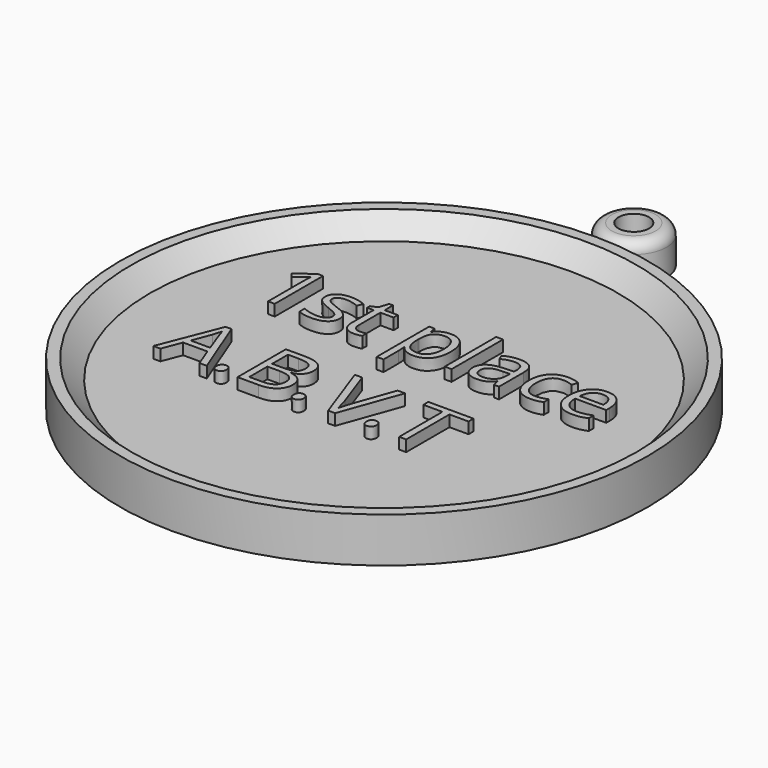
from build123d import *

# Parameters (mm, degrees)
F0_R         = 44.7882725857
F0_R_2       = 37.8315879498
F1_DEPTH     = 7.62
F0_R_3       = 5.569727431
F0_R_4       = 2.5947856339
F2_DEPTH     = 6.35
F3_R         = 1.8396307345
F0_W         = 1.1629488242
F0_H         = 10.8967632599
F4_DEPTH     = 4.445
F0_TEXT_SIZE = 14.3407947487
F5_DEPTH     = 6.35


# Not quite as in the source:
# - a fillet or chamfer that OpenCascade refuses, or shapes differently, is made with other operations: its cross-section is extruded or revolved along the edge and cut away or added
# - Text() gives the source's letters only with a copy of the font that has no kerning and outlines rounded to 1/6400 em; it was checked with that copy


with BuildPart() as f1:
    # F0 (on Top) → F1 (new body)
    with BuildSketch(Plane.XY):
        with Locations((-31.6393449903, -5.1120719872)):
            Circle(F0_R)
        with Locations((-31.6393449903, -5.1120719872)):
            Circle(F0_R_2, mode=Mode.SUBTRACT)
    extrude(amount=F1_DEPTH)

    # F0 (on Top) → F4 (join)
    with BuildSketch(Plane.XY):
        with Locations((-31.6393449903, -5.1120719872)):
            Circle(F0_R_2)
        Polygon((-50.1972631189, -19.5034808583), (-51.4296751676, -19.5034808583), (-52.7046614508, -16.2476723005), (-56.8074731984, -16.2476723005), (-58.0667742373, -19.5034808583), (-59.2722972958, -19.5034808583), (-55.2255042777, -9.2229236228), (-54.2238893945, -9.2229236228), align=None, mode=Mode.SUBTRACT)
        with BuildLine():
            add(Edge.make_bspline(
                [(-48.8987489694, -19.4866752394), (-49.1329072587, -19.2659614452), (-49.1329072587, -18.7617928799)],
                knots=[0, 0, 0, 1, 1, 1], degree=2))
            add(Edge.make_bspline(
                [(-49.1329072587, -18.7617928799), (-49.1329072587, -18.2912355522), (-48.918915712, -18.0503550154)],
                knots=[0, 0, 0, 1, 1, 1], degree=2))
            add(Edge.make_bspline(
                [(-48.918915712, -18.0503550154), (-48.7049241654, -17.8094744786), (-48.3060708114, -17.8094744786)],
                knots=[0, 0, 0, 1, 1, 1], degree=2))
            add(Edge.make_bspline(
                [(-48.3060708114, -17.8094744786), (-47.9004952099, -17.8094744786), (-47.6730591682, -18.0503550154)],
                knots=[0, 0, 0, 1, 1, 1], degree=2))
            add(Edge.make_bspline(
                [(-47.6730591682, -18.0503550154), (-47.4456231265, -18.2912355522), (-47.4456231265, -18.7617928799)],
                knots=[0, 0, 0, 1, 1, 1], degree=2))
            add(Edge.make_bspline(
                [(-47.4456231265, -18.7617928799), (-47.4456231265, -19.2166649633), (-47.676420292, -19.4620269985)],
                knots=[0, 0, 0, 1, 1, 1], degree=2))
            add(Edge.make_bspline(
                [(-47.676420292, -19.4620269985), (-47.9072174575, -19.7073890336), (-48.3060708114, -19.7073890336)],
                knots=[0, 0, 0, 1, 1, 1], degree=2))
            add(Edge.make_bspline(
                [(-48.3060708114, -19.7073890336), (-48.6645906801, -19.7073890336), (-48.8987489694, -19.4866752394)],
                knots=[0, 0, 0, 1, 1, 1], degree=2))
        make_face(mode=Mode.SUBTRACT)
        with BuildLine():
            add(Edge.make_bspline(
                [(-35.7903662694, -19.4866752394), (-36.0245245586, -19.2659614452), (-36.0245245586, -18.7617928799)],
                knots=[0, 0, 0, 1, 1, 1], degree=2))
            add(Edge.make_bspline(
                [(-36.0245245586, -18.7617928799), (-36.0245245586, -18.2912355522), (-35.810533012, -18.0503550154)],
                knots=[0, 0, 0, 1, 1, 1], degree=2))
            add(Edge.make_bspline(
                [(-35.810533012, -18.0503550154), (-35.5965414654, -17.8094744786), (-35.1976881114, -17.8094744786)],
                knots=[0, 0, 0, 1, 1, 1], degree=2))
            add(Edge.make_bspline(
                [(-35.1976881114, -17.8094744786), (-34.7921125099, -17.8094744786), (-34.5646764682, -18.0503550154)],
                knots=[0, 0, 0, 1, 1, 1], degree=2))
            add(Edge.make_bspline(
                [(-34.5646764682, -18.0503550154), (-34.3372404265, -18.2912355522), (-34.3372404265, -18.7617928799)],
                knots=[0, 0, 0, 1, 1, 1], degree=2))
            add(Edge.make_bspline(
                [(-34.3372404265, -18.7617928799), (-34.3372404265, -19.2166649633), (-34.568037592, -19.4620269985)],
                knots=[0, 0, 0, 1, 1, 1], degree=2))
            add(Edge.make_bspline(
                [(-34.568037592, -19.4620269985), (-34.7988347575, -19.7073890336), (-35.1976881114, -19.7073890336)],
                knots=[0, 0, 0, 1, 1, 1], degree=2))
            add(Edge.make_bspline(
                [(-35.1976881114, -19.7073890336), (-35.5562079801, -19.7073890336), (-35.7903662694, -19.4866752394)],
                knots=[0, 0, 0, 1, 1, 1], degree=2))
        make_face(mode=Mode.SUBTRACT)
        with BuildLine():
            Line((-44.9740767815, -19.5034808583), (-44.9740767815, -9.2654978572))
            Line((-44.9740767815, -9.2654978572), (-42.0812695908, -9.2654978572))
            add(Edge.make_bspline(
                [(-42.0812695908, -9.2654978572), (-40.0444285866, -9.2654978572), (-39.1335640452, -9.874981634)],
                knots=[0, 0, 0, 1, 1, 1], degree=2))
            add(Edge.make_bspline(
                [(-39.1335640452, -9.874981634), (-38.2226995037, -10.4844654108), (-38.2226995037, -11.7997851792)],
                knots=[0, 0, 0, 1, 1, 1], degree=2))
            add(Edge.make_bspline(
                [(-38.2226995037, -11.7997851792), (-38.2226995037, -12.7117700952), (-38.7302291929, -13.3033278786)],
                knots=[0, 0, 0, 1, 1, 1], degree=2))
            add(Edge.make_bspline(
                [(-38.7302291929, -13.3033278786), (-39.237758882, -13.894885662), (-40.2124847751, -14.069664098)],
                knots=[0, 0, 0, 1, 1, 1], degree=2))
            Line((-40.2124847751, -14.069664098), (-40.2124847751, -14.1391273226))
            add(Edge.make_bspline(
                [(-40.2124847751, -14.1391273226), (-37.8798648793, -14.5379806765), (-37.8798648793, -16.5905069249)],
                knots=[0, 0, 0, 1, 1, 1], degree=2))
            add(Edge.make_bspline(
                [(-37.8798648793, -16.5905069249), (-37.8798648793, -17.9618454228), (-38.8075350396, -18.7326631405)],
                knots=[0, 0, 0, 1, 1, 1], degree=2))
            add(Edge.make_bspline(
                [(-38.8075350396, -18.7326631405), (-39.7352051999, -19.5034808583), (-41.4023225894, -19.5034808583)],
                knots=[0, 0, 0, 1, 1, 1], degree=2))
            Line((-41.4023225894, -19.5034808583), (-44.9740767815, -19.5034808583))
        make_face(mode=Mode.SUBTRACT)
        with BuildLine():
            add(Edge.make_bspline(
                [(-23.439356792, -19.4866752394), (-23.6735150813, -19.2659614452), (-23.6735150813, -18.7617928799)],
                knots=[0, 0, 0, 1, 1, 1], degree=2))
            add(Edge.make_bspline(
                [(-23.6735150813, -18.7617928799), (-23.6735150813, -18.2912355522), (-23.4595235347, -18.0503550154)],
                knots=[0, 0, 0, 1, 1, 1], degree=2))
            add(Edge.make_bspline(
                [(-23.4595235347, -18.0503550154), (-23.245531988, -17.8094744786), (-22.8466786341, -17.8094744786)],
                knots=[0, 0, 0, 1, 1, 1], degree=2))
            add(Edge.make_bspline(
                [(-22.8466786341, -17.8094744786), (-22.4411030326, -17.8094744786), (-22.2136669909, -18.0503550154)],
                knots=[0, 0, 0, 1, 1, 1], degree=2))
            add(Edge.make_bspline(
                [(-22.2136669909, -18.0503550154), (-21.9862309491, -18.2912355522), (-21.9862309491, -18.7617928799)],
                knots=[0, 0, 0, 1, 1, 1], degree=2))
            add(Edge.make_bspline(
                [(-21.9862309491, -18.7617928799), (-21.9862309491, -19.2166649633), (-22.2170281146, -19.4620269985)],
                knots=[0, 0, 0, 1, 1, 1], degree=2))
            add(Edge.make_bspline(
                [(-22.2170281146, -19.4620269985), (-22.4478252801, -19.7073890336), (-22.8466786341, -19.7073890336)],
                knots=[0, 0, 0, 1, 1, 1], degree=2))
            add(Edge.make_bspline(
                [(-22.8466786341, -19.7073890336), (-23.2051985028, -19.7073890336), (-23.439356792, -19.4866752394)],
                knots=[0, 0, 0, 1, 1, 1], degree=2))
        make_face(mode=Mode.SUBTRACT)
        with BuildLine():
            Line((-28.3566808664, -15.8488189465), (-26.017338723, -9.2654978572))
            Line((-26.017338723, -9.2654978572), (-24.7378709416, -9.2654978572))
            Line((-24.7378709416, -9.2654978572), (-28.426144091, -19.5034808583))
            Line((-28.426144091, -19.5034808583), (-29.6025374102, -19.5034808583))
            Line((-29.6025374102, -19.5034808583), (-33.2728845662, -9.2654978572))
            Line((-33.2728845662, -9.2654978572), (-32.0113427782, -9.2654978572))
            Line((-32.0113427782, -9.2654978572), (-29.6585561397, -15.8891524318))
            add(Edge.make_bspline(
                [(-29.6585561397, -15.8891524318), (-29.2529805382, -17.0319345133), (-29.0154611252, -18.1097348686)],
                knots=[0, 0, 0, 1, 1, 1], degree=2))
            add(Edge.make_bspline(
                [(-29.0154611252, -18.1097348686), (-28.7622564679, -16.9759157838), (-28.3566808664, -15.8488189465)],
                knots=[0, 0, 0, 1, 1, 1], degree=2))
        make_face(mode=Mode.SUBTRACT)
        Polygon((-16.3641912578, -10.3231314699), (-16.3641912578, -19.5034808583), (-17.5540290721, -19.5034808583), (-17.5540290721, -10.3231314699), (-20.7963931348, -10.3231314699), (-20.7963931348, -9.2654978572), (-13.1218271951, -9.2654978572), (-13.1218271951, -10.3231314699), align=None, mode=Mode.SUBTRACT)
        with BuildLine():
            Line((-54.2664636289, 10.2379830011), (-54.2664636289, 0))
            Line((-54.2664636289, 0), (-55.4002827137, 0))
            Line((-55.4002827137, 0), (-55.4002827137, 7.2958793284))
            add(Edge.make_bspline(
                [(-55.4002827137, 7.2958793284), (-55.4002827137, 8.2078642445), (-55.3442639842, 9.0190154474)],
                knots=[0, 0, 0, 1, 1, 1], degree=2))
            add(Edge.make_bspline(
                [(-55.3442639842, 9.0190154474), (-55.4899126809, 8.8711260016), (-55.672533739, 8.7109124353)],
                knots=[0, 0, 0, 1, 1, 1], degree=2))
            add(Edge.make_bspline(
                [(-55.672533739, 8.7109124353), (-55.8551547971, 8.5506988689), (-57.3385307539, 7.3451758104)],
                knots=[0, 0, 0, 1, 1, 1], degree=2))
            Line((-57.3385307539, 7.3451758104), (-57.9547367783, 8.1428825183))
            Line((-57.9547367783, 8.1428825183), (-55.2456710203, 10.2379830011))
            Line((-55.2456710203, 10.2379830011), (-54.2664636289, 10.2379830011))
        make_face(mode=Mode.SUBTRACT)
        with BuildLine():
            add(Edge.make_bspline(
                [(-45.3706893863, 3.3611237692), (-44.8911690619, 2.8569552038), (-44.8911690619, 2.0928597336)],
                knots=[0, 0, 0, 1, 1, 1], degree=2))
            add(Edge.make_bspline(
                [(-44.8911690619, 2.0928597336), (-44.8911690619, 1.0217816258), (-45.6888757698, 0.4403072138)],
                knots=[0, 0, 0, 1, 1, 1], degree=2))
            add(Edge.make_bspline(
                [(-45.6888757698, 0.4403072138), (-46.4865824777, -0.1411671983), (-47.9296249493, -0.1411671983)],
                knots=[0, 0, 0, 1, 1, 1], degree=2))
            add(Edge.make_bspline(
                [(-47.9296249493, -0.1411671983), (-49.4555751405, -0.1411671983), (-50.3093005779, 0.3428346245)],
                knots=[0, 0, 0, 1, 1, 1], degree=2))
            Line((-50.3093005779, 0.3428346245), (-50.3093005779, 1.4206349798))
            add(Edge.make_bspline(
                [(-50.3093005779, 1.4206349798), (-49.7558355306, 1.1405413324), (-49.1228238873, 0.980327766)],
                knots=[0, 0, 0, 1, 1, 1], degree=2))
            add(Edge.make_bspline(
                [(-49.1228238873, 0.980327766), (-48.4898122441, 0.8201141997), (-47.9004952099, 0.8201141997)],
                knots=[0, 0, 0, 1, 1, 1], degree=2))
            add(Edge.make_bspline(
                [(-47.9004952099, 0.8201141997), (-46.9907510431, 0.8201141997), (-46.5011473473, 1.1102912184)],
                knots=[0, 0, 0, 1, 1, 1], degree=2))
            add(Edge.make_bspline(
                [(-46.5011473473, 1.1102912184), (-46.0115436516, 1.4004682372), (-46.0115436516, 1.9965075189)],
                knots=[0, 0, 0, 1, 1, 1], degree=2))
            add(Edge.make_bspline(
                [(-46.0115436516, 1.9965075189), (-46.0115436516, 2.4446573548), (-46.3991932597, 2.7628437383)],
                knots=[0, 0, 0, 1, 1, 1], degree=2))
            add(Edge.make_bspline(
                [(-46.3991932597, 2.7628437383), (-46.7868428677, 3.0810301218), (-47.9161804542, 3.5157354626)],
                knots=[0, 0, 0, 1, 1, 1], degree=2))
            add(Edge.make_bspline(
                [(-47.9161804542, 3.5157354626), (-48.987258562, 3.9145888166), (-49.4387695217, 4.2126084574)],
                knots=[0, 0, 0, 1, 1, 1], degree=2))
            add(Edge.make_bspline(
                [(-49.4387695217, 4.2126084574), (-49.8902804813, 4.5106280983), (-50.1109942755, 4.8881943351)],
                knots=[0, 0, 0, 1, 1, 1], degree=2))
            add(Edge.make_bspline(
                [(-50.1109942755, 4.8881943351), (-50.3317080697, 5.2657605718), (-50.3317080697, 5.7900958798)],
                knots=[0, 0, 0, 1, 1, 1], degree=2))
            add(Edge.make_bspline(
                [(-50.3317080697, 5.7900958798), (-50.3317080697, 6.728969786), (-49.5676125995, 7.272351462)],
                knots=[0, 0, 0, 1, 1, 1], degree=2))
            add(Edge.make_bspline(
                [(-49.5676125995, 7.272351462), (-48.8035171293, 7.8157331381), (-47.4747528658, 7.8157331381)],
                knots=[0, 0, 0, 1, 1, 1], degree=2))
            add(Edge.make_bspline(
                [(-47.4747528658, 7.8157331381), (-46.2356185696, 7.8157331381), (-45.0502622536, 7.3115645727)],
                knots=[0, 0, 0, 1, 1, 1], degree=2))
            Line((-45.0502622536, 7.3115645727), (-45.4648008518, 6.3659684189))
            add(Edge.make_bspline(
                [(-45.4648008518, 6.3659684189), (-46.6187866793, 6.841007245), (-47.5576605855, 6.841007245)],
                knots=[0, 0, 0, 1, 1, 1], degree=2))
            add(Edge.make_bspline(
                [(-47.5576605855, 6.841007245), (-48.3844970327, 6.841007245), (-48.8046375039, 6.5822007147)],
                knots=[0, 0, 0, 1, 1, 1], degree=2))
            add(Edge.make_bspline(
                [(-48.8046375039, 6.5822007147), (-49.224777975, 6.3233941845), (-49.224777975, 5.8685221011)],
                knots=[0, 0, 0, 1, 1, 1], degree=2))
            add(Edge.make_bspline(
                [(-49.224777975, 5.8685221011), (-49.224777975, 5.5592987143), (-49.0668051579, 5.3430664185)],
                knots=[0, 0, 0, 1, 1, 1], degree=2))
            add(Edge.make_bspline(
                [(-49.0668051579, 5.3430664185), (-48.9088323407, 5.1268341227), (-48.5592754687, 4.9307685695)],
                knots=[0, 0, 0, 1, 1, 1], degree=2))
            add(Edge.make_bspline(
                [(-48.5592754687, 4.9307685695), (-48.2097185967, 4.7347030163), (-47.214825961, 4.3627386525)],
                knots=[0, 0, 0, 1, 1, 1], degree=2))
            add(Edge.make_bspline(
                [(-47.214825961, 4.3627386525), (-45.8502097107, 3.8652923346), (-45.3706893863, 3.3611237692)],
                knots=[0, 0, 0, 1, 1, 1], degree=2))
        make_face(mode=Mode.SUBTRACT)
        with BuildLine():
            add(Edge.make_bspline(
                [(-41.4247300812, 1.1909581889), (-41.0953399518, 0.8201141997), (-40.5217081619, 0.8201141997)],
                knots=[0, 0, 0, 1, 1, 1], degree=2))
            add(Edge.make_bspline(
                [(-40.5217081619, 0.8201141997), (-40.2124847751, 0.8201141997), (-39.9256688801, 0.8649291833)],
                knots=[0, 0, 0, 1, 1, 1], degree=2))
            add(Edge.make_bspline(
                [(-39.9256688801, 0.8649291833), (-39.6388529852, 0.9097441669), (-39.4707967967, 0.9590406488)],
                knots=[0, 0, 0, 1, 1, 1], degree=2))
            Line((-39.4707967967, 0.9590406488), (-39.4707967967, 0.0694632246))
            add(Edge.make_bspline(
                [(-39.4707967967, 0.0694632246), (-39.6590197278, -0.0201667426), (-40.0265025932, -0.0806669705)],
                knots=[0, 0, 0, 1, 1, 1], degree=2))
            add(Edge.make_bspline(
                [(-40.0265025932, -0.0806669705), (-40.3939854586, -0.1411671983), (-40.6897643503, -0.1411671983)],
                knots=[0, 0, 0, 1, 1, 1], degree=2))
            add(Edge.make_bspline(
                [(-40.6897643503, -0.1411671983), (-42.9148282856, -0.1411671983), (-42.9148282856, 2.2048971926)],
                knots=[0, 0, 0, 1, 1, 1], degree=2))
            Line((-42.9148282856, 2.2048971926), (-42.9148282856, 6.7715440204))
            Line((-42.9148282856, 6.7715440204), (-44.0150361327, 6.7715440204))
            Line((-44.0150361327, 6.7715440204), (-44.0150361327, 7.3317313153))
            Line((-44.0150361327, 7.3317313153), (-42.9148282856, 7.8157331381))
            Line((-42.9148282856, 7.8157331381), (-42.4263449644, 9.4537207883))
            Line((-42.4263449644, 9.4537207883), (-41.7541202106, 9.4537207883))
            Line((-41.7541202106, 9.4537207883), (-41.7541202106, 7.6745659398))
            Line((-41.7541202106, 7.6745659398), (-39.5268155262, 7.6745659398))
            Line((-39.5268155262, 7.6745659398), (-39.5268155262, 6.7715440204))
            Line((-39.5268155262, 6.7715440204), (-41.7541202106, 6.7715440204))
            Line((-41.7541202106, 6.7715440204), (-41.7541202106, 2.2541936746))
            add(Edge.make_bspline(
                [(-41.7541202106, 2.2541936746), (-41.7541202106, 1.5618021781), (-41.4247300812, 1.1909581889)],
                knots=[0, 0, 0, 1, 1, 1], degree=2))
        make_face(mode=Mode.SUBTRACT)
        with BuildLine():
            add(Edge.make_bspline(
                [(-28.2973010132, 0.9063830431), (-29.1409430793, -0.1411671983), (-30.6400042803, -0.1411671983)],
                knots=[0, 0, 0, 1, 1, 1], degree=2))
            add(Edge.make_bspline(
                [(-30.6400042803, -0.1411671983), (-31.3906552555, -0.1411671983), (-32.0102224036, 0.1355653254)],
                knots=[0, 0, 0, 1, 1, 1], degree=2))
            add(Edge.make_bspline(
                [(-32.0102224036, 0.1355653254), (-32.6297895517, 0.412297849), (-33.0488096483, 0.9881703882)],
                knots=[0, 0, 0, 1, 1, 1], degree=2))
            Line((-33.0488096483, 0.9881703882), (-33.1339581171, 0.9881703882))
            add(Edge.make_bspline(
                [(-33.1339581171, 0.9881703882), (-33.0488096483, 0.3159456343), (-33.0488096483, -0.286815895)],
                knots=[0, 0, 0, 1, 1, 1], degree=2))
            Line((-33.0488096483, -0.286815895), (-33.0488096483, -3.4462722381))
            Line((-33.0488096483, -3.4462722381), (-34.2117584724, -3.4462722381))
            Line((-34.2117584724, -3.4462722381), (-34.2117584724, 7.6745659398))
            Line((-34.2117584724, 7.6745659398), (-33.2661623187, 7.6745659398))
            Line((-33.2661623187, 7.6745659398), (-33.1048283778, 6.6236545746))
            Line((-33.1048283778, 6.6236545746), (-33.0488096483, 6.6236545746))
            add(Edge.make_bspline(
                [(-33.0488096483, 6.6236545746), (-32.6006598124, 7.2555458432), (-32.0057409052, 7.5356394906)],
                knots=[0, 0, 0, 1, 1, 1], degree=2))
            add(Edge.make_bspline(
                [(-32.0057409052, 7.5356394906), (-31.4108219981, 7.8157331381), (-30.6400042803, 7.8157331381)],
                knots=[0, 0, 0, 1, 1, 1], degree=2))
            add(Edge.make_bspline(
                [(-30.6400042803, 7.8157331381), (-29.1140540891, 7.8157331381), (-28.2838565181, 6.7715440204)],
                knots=[0, 0, 0, 1, 1, 1], degree=2))
            add(Edge.make_bspline(
                [(-28.2838565181, 6.7715440204), (-27.4536589471, 5.7273549028), (-27.4536589471, 3.845125592)],
                knots=[0, 0, 0, 1, 1, 1], degree=2))
            add(Edge.make_bspline(
                [(-27.4536589471, 3.845125592), (-27.4536589471, 1.9539332845), (-28.2973010132, 0.9063830431)],
                knots=[0, 0, 0, 1, 1, 1], degree=2))
        make_face(mode=Mode.SUBTRACT)
        with Locations((-24.8420657784, 5.4483816299)):
            Rectangle(F0_W, F0_H, mode=Mode.SUBTRACT)
        with BuildLine():
            Line((-16.2140610628, 0), (-17.0767494969, 0))
            Line((-17.0767494969, 0), (-17.3075466624, 1.0934855996))
            Line((-17.3075466624, 1.0934855996), (-17.3635653919, 1.0934855996))
            add(Edge.make_bspline(
                [(-17.3635653919, 1.0934855996), (-17.9371971818, 0.3719643638), (-18.507467848, 0.1153985827)],
                knots=[0, 0, 0, 1, 1, 1], degree=2))
            add(Edge.make_bspline(
                [(-18.507467848, 0.1153985827), (-19.0777385142, -0.1411671983), (-19.9337047007, -0.1411671983)],
                knots=[0, 0, 0, 1, 1, 1], degree=2))
            add(Edge.make_bspline(
                [(-19.9337047007, -0.1411671983), (-21.0742460331, -0.1411671983), (-21.721822546, 0.4481498359)],
                knots=[0, 0, 0, 1, 1, 1], degree=2))
            add(Edge.make_bspline(
                [(-21.721822546, 0.4481498359), (-22.3693990588, 1.0374668701), (-22.3693990588, 2.121989473)],
                knots=[0, 0, 0, 1, 1, 1], degree=2))
            add(Edge.make_bspline(
                [(-22.3693990588, 2.121989473), (-22.3693990588, 4.4456463721), (-18.6519961701, 4.5576838311)],
                knots=[0, 0, 0, 1, 1, 1], degree=2))
            Line((-18.6519961701, 4.5576838311), (-17.3501208968, 4.6002580655))
            Line((-17.3501208968, 4.6002580655), (-17.3501208968, 5.0775376407))
            add(Edge.make_bspline(
                [(-17.3501208968, 5.0775376407), (-17.3501208968, 5.9805595601), (-17.7377705048, 6.4107834025)],
                knots=[0, 0, 0, 1, 1, 1], degree=2))
            add(Edge.make_bspline(
                [(-17.7377705048, 6.4107834025), (-18.1254201129, 6.841007245), (-18.9813862995, 6.841007245)],
                knots=[0, 0, 0, 1, 1, 1], degree=2))
            add(Edge.make_bspline(
                [(-18.9813862995, 6.841007245), (-19.9404269483, 6.841007245), (-21.1504315052, 6.25393096)],
                knots=[0, 0, 0, 1, 1, 1], degree=2))
            Line((-21.1504315052, 6.25393096), (-21.5089513739, 7.1435083842))
            add(Edge.make_bspline(
                [(-21.5089513739, 7.1435083842), (-20.9420418315, 7.4504910218), (-20.2664559539, 7.6252694578)],
                knots=[0, 0, 0, 1, 1, 1], degree=2))
            add(Edge.make_bspline(
                [(-20.2664559539, 7.6252694578), (-19.5908700763, 7.8000478938), (-18.9096823257, 7.8000478938)],
                knots=[0, 0, 0, 1, 1, 1], degree=2))
            add(Edge.make_bspline(
                [(-18.9096823257, 7.8000478938), (-17.5383438279, 7.8000478938), (-16.8762024453, 7.1916844916)],
                knots=[0, 0, 0, 1, 1, 1], degree=2))
            add(Edge.make_bspline(
                [(-16.8762024453, 7.1916844916), (-16.2140610628, 6.5833210893), (-16.2140610628, 5.2388715816)],
                knots=[0, 0, 0, 1, 1, 1], degree=2))
            Line((-16.2140610628, 5.2388715816), (-16.2140610628, 0))
        make_face(mode=Mode.SUBTRACT)
        with BuildLine():
            add(Edge.make_bspline(
                [(-8.8151072721, 0.2599269048), (-9.5836842407, -0.1411671983), (-10.7533553124, -0.1411671983)],
                knots=[0, 0, 0, 1, 1, 1], degree=2))
            add(Edge.make_bspline(
                [(-10.7533553124, -0.1411671983), (-12.4204727019, -0.1411671983), (-13.3346983671, 0.8850959259)],
                knots=[0, 0, 0, 1, 1, 1], degree=2))
            add(Edge.make_bspline(
                [(-13.3346983671, 0.8850959259), (-14.2489240324, 1.9113590501), (-14.2489240324, 3.7891068625)],
                knots=[0, 0, 0, 1, 1, 1], degree=2))
            add(Edge.make_bspline(
                [(-14.2489240324, 3.7891068625), (-14.2489240324, 5.7139104077), (-13.3201334975, 6.7648217729)],
                knots=[0, 0, 0, 1, 1, 1], degree=2))
            add(Edge.make_bspline(
                [(-13.3201334975, 6.7648217729), (-12.3913429626, 7.8157331381), (-10.6771698403, 7.8157331381)],
                knots=[0, 0, 0, 1, 1, 1], degree=2))
            add(Edge.make_bspline(
                [(-10.6771698403, 7.8157331381), (-10.1237047929, 7.8157331381), (-9.5702397456, 7.695853057)],
                knots=[0, 0, 0, 1, 1, 1], degree=2))
            add(Edge.make_bspline(
                [(-9.5702397456, 7.695853057), (-9.0167746983, 7.5759729759), (-8.7030698131, 7.4146390349)],
                knots=[0, 0, 0, 1, 1, 1], degree=2))
            Line((-8.7030698131, 7.4146390349), (-9.0593489327, 6.428709396))
            add(Edge.make_bspline(
                [(-9.0593489327, 6.428709396), (-9.4447577915, 6.5833210893), (-9.899629875, 6.6841548024)],
                knots=[0, 0, 0, 1, 1, 1], degree=2))
            add(Edge.make_bspline(
                [(-9.899629875, 6.6841548024), (-10.3545019584, 6.7849885155), (-10.7040588304, 6.7849885155)],
                knots=[0, 0, 0, 1, 1, 1], degree=2))
            add(Edge.make_bspline(
                [(-10.7040588304, 6.7849885155), (-13.0434009738, 6.7849885155), (-13.0434009738, 3.8025513576)],
                knots=[0, 0, 0, 1, 1, 1], degree=2))
            add(Edge.make_bspline(
                [(-13.0434009738, 3.8025513576), (-13.0434009738, 2.3886386253), (-12.4731303076, 1.6323857773)],
                knots=[0, 0, 0, 1, 1, 1], degree=2))
            add(Edge.make_bspline(
                [(-12.4731303076, 1.6323857773), (-11.9028596414, 0.8761329292), (-10.7824850517, 0.8761329292)],
                knots=[0, 0, 0, 1, 1, 1], degree=2))
            add(Edge.make_bspline(
                [(-10.7824850517, 0.8761329292), (-9.8234444029, 0.8761329292), (-8.8151072721, 1.2884307782)],
                knots=[0, 0, 0, 1, 1, 1], degree=2))
            Line((-8.8151072721, 1.2884307782), (-8.8151072721, 0.2599269048))
        make_face(mode=Mode.SUBTRACT)
        with BuildLine():
            add(Edge.make_bspline(
                [(-2.4244906122, -0.024648241), (-2.9734741612, -0.1411671983), (-3.7510141265, -0.1411671983)],
                knots=[0, 0, 0, 1, 1, 1], degree=2))
            add(Edge.make_bspline(
                [(-3.7510141265, -0.1411671983), (-5.4517427537, -0.1411671983), (-6.4365520181, 0.8962996718)],
                knots=[0, 0, 0, 1, 1, 1], degree=2))
            add(Edge.make_bspline(
                [(-6.4365520181, 0.8962996718), (-7.4213612825, 1.9337665419), (-7.4213612825, 3.7734216183)],
                knots=[0, 0, 0, 1, 1, 1], degree=2))
            add(Edge.make_bspline(
                [(-7.4213612825, 3.7734216183), (-7.4213612825, 5.6310026881), (-6.5071356172, 6.7233679131)],
                knots=[0, 0, 0, 1, 1, 1], degree=2))
            add(Edge.make_bspline(
                [(-6.5071356172, 6.7233679131), (-5.592909952, 7.8157331381), (-4.0512745165, 7.8157331381)],
                knots=[0, 0, 0, 1, 1, 1], degree=2))
            add(Edge.make_bspline(
                [(-4.0512745165, 7.8157331381), (-2.6104727941, 7.8157331381), (-1.7701918518, 6.8667758605)],
                knots=[0, 0, 0, 1, 1, 1], degree=2))
            add(Edge.make_bspline(
                [(-1.7701918518, 6.8667758605), (-0.9299109095, 5.917818583), (-0.9299109095, 4.3627386525)],
                knots=[0, 0, 0, 1, 1, 1], degree=2))
            Line((-0.9299109095, 4.3627386525), (-0.9299109095, 3.6277729216))
            Line((-0.9299109095, 3.6277729216), (-6.2158382239, 3.6277729216))
            add(Edge.make_bspline(
                [(-6.2158382239, 3.6277729216), (-6.179986237, 2.2766011664), (-5.5324097242, 1.5763670478)],
                knots=[0, 0, 0, 1, 1, 1], degree=2))
            add(Edge.make_bspline(
                [(-5.5324097242, 1.5763670478), (-4.8848332113, 0.8761329292), (-3.7084398921, 0.8761329292)],
                knots=[0, 0, 0, 1, 1, 1], degree=2))
            add(Edge.make_bspline(
                [(-3.7084398921, 0.8761329292), (-2.4693055958, 0.8761329292), (-1.2593010389, 1.3937459896)],
                knots=[0, 0, 0, 1, 1, 1], degree=2))
            Line((-1.2593010389, 1.3937459896), (-1.2593010389, 0.3562791195))
            add(Edge.make_bspline(
                [(-1.2593010389, 0.3562791195), (-1.8755070632, 0.0918707164), (-2.4244906122, -0.024648241)],
                knots=[0, 0, 0, 1, 1, 1], degree=2))
        make_face(mode=Mode.SUBTRACT)
    extrude(amount=F4_DEPTH)

    # F6: chamfer of 5.08 on 1 edges, made by hand


with BuildPart() as f2:
    # F0 (on Top) → F2 (new body)
    with BuildSketch(Plane.XY):
        with Locations((-31.6393449903, 47.8641353548)):
            Circle(F0_R_3)
        with Locations((-31.6393449903, 47.8641353548)):
            Circle(F0_R_4, mode=Mode.SUBTRACT)
    extrude(amount=F2_DEPTH)

    # F3
    f3_edges = [f2.edges().sort_by_distance(p)[0] for p in [
        (-37.209072, 47.864135, 6.35),
    ]]
    fillet(f3_edges, radius=F3_R)


with BuildPart() as f4:
    # F0 (on Top) → F4, piece 2 (new body)
    with BuildSketch(Plane.XY):
        with BuildLine():
            Line((-56.3862123527, -15.1765941927), (-53.0743850654, -15.1765941927))
            Line((-53.0743850654, -15.1765941927), (-54.2664636289, -12.0036933545))
            add(Edge.make_bspline(
                [(-54.2664636289, -12.0036933545), (-54.4972607944, -11.4009318252), (-54.7415024549, -10.5270396452)],
                knots=[0, 0, 0, 1, 1, 1], degree=2))
            add(Edge.make_bspline(
                [(-54.7415024549, -10.5270396452), (-54.8961141483, -11.1992643991), (-55.1829300433, -12.0036933545)],
                knots=[0, 0, 0, 1, 1, 1], degree=2))
            Line((-55.1829300433, -12.0036933545), (-56.3862123527, -15.1765941927))
        make_face()
    extrude(amount=F4_DEPTH)


with BuildPart() as f4b:
    # F0 (on Top) → F4, piece 3 (new body)
    with BuildSketch(Plane.XY):
        with BuildLine():
            Line((-41.7451572139, -14.656740383), (-43.7842389672, -14.656740383))
            Line((-43.7842389672, -14.656740383), (-43.7842389672, -18.48842148))
            Line((-43.7842389672, -18.48842148), (-41.64656425, -18.48842148))
            add(Edge.make_bspline(
                [(-41.64656425, -18.48842148), (-40.4074299537, -18.48842148), (-39.7811405581, -18.0089011556)],
                knots=[0, 0, 0, 1, 1, 1], degree=2))
            add(Edge.make_bspline(
                [(-39.7811405581, -18.0089011556), (-39.1548511624, -17.5293808311), (-39.1548511624, -16.5053584561)],
                knots=[0, 0, 0, 1, 1, 1], degree=2))
            add(Edge.make_bspline(
                [(-39.1548511624, -16.5053584561), (-39.1548511624, -15.5530400548), (-39.7957054277, -15.1048902189)],
                knots=[0, 0, 0, 1, 1, 1], degree=2))
            add(Edge.make_bspline(
                [(-39.7957054277, -15.1048902189), (-40.4365596931, -14.656740383), (-41.7451572139, -14.656740383)],
                knots=[0, 0, 0, 1, 1, 1], degree=2))
        make_face()
    extrude(amount=F4_DEPTH)


with BuildPart() as f4c:
    # F0 (on Top) → F4, piece 4 (new body)
    with BuildSketch(Plane.XY):
        with BuildLine():
            Line((-43.7842389672, -10.2962424798), (-43.7842389672, -13.6484032523))
            Line((-43.7842389672, -13.6484032523), (-41.8235834352, -13.6484032523))
            add(Edge.make_bspline(
                [(-41.8235834352, -13.6484032523), (-40.5620416471, -13.6484032523), (-40.0085765998, -13.2529110221)],
                knots=[0, 0, 0, 1, 1, 1], degree=2))
            add(Edge.make_bspline(
                [(-40.0085765998, -13.2529110221), (-39.4551115524, -12.8574187919), (-39.4551115524, -11.9207856349)],
                knots=[0, 0, 0, 1, 1, 1], degree=2))
            add(Edge.make_bspline(
                [(-39.4551115524, -11.9207856349), (-39.4551115524, -11.0580972008), (-40.0713175768, -10.6771698403)],
                knots=[0, 0, 0, 1, 1, 1], degree=2))
            add(Edge.make_bspline(
                [(-40.0713175768, -10.6771698403), (-40.6875236012, -10.2962424798), (-42.0319731089, -10.2962424798)],
                knots=[0, 0, 0, 1, 1, 1], degree=2))
            Line((-42.0319731089, -10.2962424798), (-43.7842389672, -10.2962424798))
        make_face()
    extrude(amount=F4_DEPTH)


with BuildPart() as f4d:
    # F0 (on Top) → F4, piece 5 (new body)
    with BuildSketch(Plane.XY):
        with BuildLine():
            add(Edge.make_bspline(
                [(-29.2227304243, 6.0612265305), (-29.7862788429, 6.8275627499), (-30.8080604688, 6.8275627499)],
                knots=[0, 0, 0, 1, 1, 1], degree=2))
            add(Edge.make_bspline(
                [(-30.8080604688, 6.8275627499), (-31.984453788, 6.8275627499), (-32.5099094706, 6.1766251133)],
                knots=[0, 0, 0, 1, 1, 1], degree=2))
            add(Edge.make_bspline(
                [(-32.5099094706, 6.1766251133), (-33.0353651532, 5.5256874766), (-33.0488096483, 4.1028117476)],
                knots=[0, 0, 0, 1, 1, 1], degree=2))
            Line((-33.0488096483, 4.1028117476), (-33.0488096483, 3.845125592))
            add(Edge.make_bspline(
                [(-33.0488096483, 3.845125592), (-33.0488096483, 2.2273046844), (-32.5099094706, 1.5304316896)],
                knots=[0, 0, 0, 1, 1, 1], degree=2))
            add(Edge.make_bspline(
                [(-32.5099094706, 1.5304316896), (-31.971009293, 0.8335586948), (-30.7811714786, 0.8335586948)],
                knots=[0, 0, 0, 1, 1, 1], degree=2))
            add(Edge.make_bspline(
                [(-30.7811714786, 0.8335586948), (-29.7862788429, 0.8335586948), (-29.2227304243, 1.6391080248)],
                knots=[0, 0, 0, 1, 1, 1], degree=2))
            add(Edge.make_bspline(
                [(-29.2227304243, 1.6391080248), (-28.6591820057, 2.4446573548), (-28.6591820057, 3.8585700871)],
                knots=[0, 0, 0, 1, 1, 1], degree=2))
            add(Edge.make_bspline(
                [(-28.6591820057, 3.8585700871), (-28.6591820057, 5.2948903111), (-29.2227304243, 6.0612265305)],
                knots=[0, 0, 0, 1, 1, 1], degree=2))
        make_face()
    extrude(amount=F4_DEPTH)


with BuildPart() as f4e:
    # F0 (on Top) → F4, piece 6 (new body)
    with BuildSketch(Plane.XY):
        with BuildLine():
            add(Edge.make_bspline(
                [(-20.7695041447, 1.1483839545), (-20.3885767842, 0.8201141997), (-19.7029075352, 0.8201141997)],
                knots=[0, 0, 0, 1, 1, 1], degree=2))
            add(Edge.make_bspline(
                [(-19.7029075352, 0.8201141997), (-18.6161441832, 0.8201141997), (-17.9965770351, 1.4150331068)],
                knots=[0, 0, 0, 1, 1, 1], degree=2))
            add(Edge.make_bspline(
                [(-17.9965770351, 1.4150331068), (-17.3770098869, 2.009952014), (-17.3770098869, 3.0810301218)],
                knots=[0, 0, 0, 1, 1, 1], degree=2))
            Line((-17.3770098869, 3.0810301218), (-17.3770098869, 3.7734216183))
            Line((-17.3770098869, 3.7734216183), (-18.5399587111, 3.7263658855))
            add(Edge.make_bspline(
                [(-18.5399587111, 3.7263658855), (-19.9269824532, 3.6770694035), (-20.5387069792, 3.2950216684)],
                knots=[0, 0, 0, 1, 1, 1], degree=2))
            add(Edge.make_bspline(
                [(-20.5387069792, 3.2950216684), (-21.1504315052, 2.9129739333), (-21.1504315052, 2.1085449779)],
                knots=[0, 0, 0, 1, 1, 1], degree=2))
            add(Edge.make_bspline(
                [(-21.1504315052, 2.1085449779), (-21.1504315052, 1.4766537093), (-20.7695041447, 1.1483839545)],
                knots=[0, 0, 0, 1, 1, 1], degree=2))
        make_face()
    extrude(amount=F4_DEPTH)


with BuildPart() as f4f:
    # F0 (on Top) → F4, piece 7 (new body)
    with BuildSketch(Plane.XY):
        with BuildLine():
            add(Edge.make_bspline(
                [(-2.665371149, 6.2561717091), (-3.1549748447, 6.841007245), (-4.0669597608, 6.841007245)],
                knots=[0, 0, 0, 1, 1, 1], degree=2))
            add(Edge.make_bspline(
                [(-4.0669597608, 6.841007245), (-4.9901484227, 6.841007245), (-5.5402523463, 6.2393660903)],
                knots=[0, 0, 0, 1, 1, 1], degree=2))
            add(Edge.make_bspline(
                [(-5.5402523463, 6.2393660903), (-6.0903562699, 5.6377249356), (-6.1889492337, 4.5733690753)],
                knots=[0, 0, 0, 1, 1, 1], degree=2))
            Line((-6.1889492337, 4.5733690753), (-2.1757674533, 4.5733690753))
            add(Edge.make_bspline(
                [(-2.1757674533, 4.5733690753), (-2.1757674533, 5.6713361733), (-2.665371149, 6.2561717091)],
                knots=[0, 0, 0, 1, 1, 1], degree=2))
        make_face()
    extrude(amount=F4_DEPTH)


with BuildPart() as f5:
    # F0 (on Top) → F5 (new body)
    with BuildSketch(Plane.XY):
        with Locations((-59.2722972958, 0)):
            Text('1st place', F0_TEXT_SIZE, font='Open Sans', text_align=(TextAlign.LEFT, TextAlign.BOTTOM))
        with Locations((-59.2722972958, -19.5034808583)):
            Text('A.B.V.T', F0_TEXT_SIZE, font='Open Sans', text_align=(TextAlign.LEFT, TextAlign.BOTTOM))
    extrude(amount=F5_DEPTH)


with BuildPart() as f6_tool2:
    # F6_s3 → F6_t4 (revolve)
    with BuildSketch(Plane.XZ.offset(5.1120719872)):
        Polygon((11.2722429596, 7.62), (6.1922429596, 2.54), (6.1922429596, 7.62), align=None)
    revolve(axis=Axis((-31.6393449903, -5.1120719872, 7.62), (0, 0, 1)))

    split(bisect_by=Plane.XY.offset(4.445), keep=Keep.TOP)


with BuildPart() as f1_1:
    add(f1.part)

    # F6_t1: cut F6_tool2
    add(f6_tool2.part, mode=Mode.SUBTRACT)


solid = Compound([f2.part, f4.part, f4b.part, f4c.part, f4d.part, f4e.part, f4f.part, f5.part, f1_1.part])
